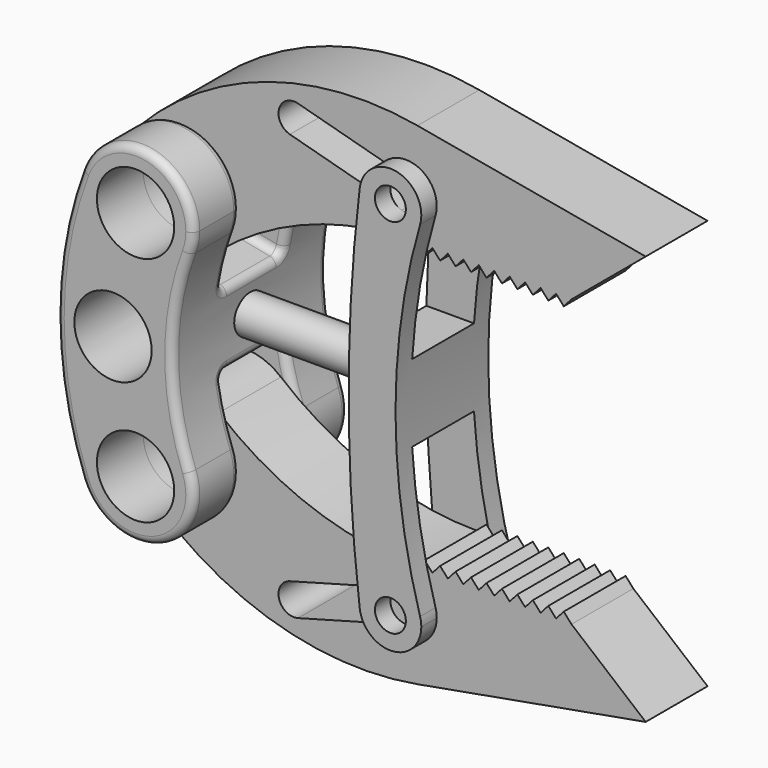
from build123d import *

# Parameters (mm, degrees)
F0_R           = 5
F2_DEPTH       = 12.5
F1_R           = 5
F3_DEPTH       = 5
F4_R           = 5
F5_DEPTH       = 25.001
F6_R           = 5
F7_DEPTH       = 5
F8_R           = 2.5
F9_DEPTH       = 60.001
F9_DEPTH_BACK  = 10.2360656985
F10_DEPTH      = 27
F10_DEPTH_BACK = 10
F11_R          = 2
F12_DEPTH      = 7.5
F14_DEPTH      = 5
F15_R          = 1


# Not quite as in the source:
# - a feature of the source that left no trace in its solid (it failed there, or was rolled back) is left out


with BuildPart() as f2:
    # F0 (on Front) → F2 (new body, symmetric)
    with BuildSketch(Plane.XZ):
        with BuildLine():
            ThreePointArc((7.0173413473, 12.3529411765), (-2.6470588235, 7.9826586527), (-7.0173413473, 17.6470588235))
            ThreePointArc((-7.0173413473, 17.6470588235), (-10.2350656985, 0), (-7.0173413473, -17.6470588235))
            ThreePointArc((-7.0173413473, -17.6470588235), (-2.6470588235, -7.9826586527), (7.0173413473, -12.3529411765))
            ThreePointArc((7.0173413473, -12.3529411765), (4.7649343015, 0), (7.0173413473, 12.3529411765))
        make_face()
        with BuildLine():
            ThreePointArc((7.5, 15), (1.3453512358, 22.3783487348), (-7.0173413473, 17.6470588235))
            ThreePointArc((-7.0173413473, 17.6470588235), (-2.6470588235, 7.9826586527), (7.0173413473, 12.3529411765))
            ThreePointArc((7.0173413473, 12.3529411765), (7.3783487348, 13.6546487642), (7.5, 15))
        make_face()
        with Locations((0, 15)):
            Circle(F0_R, mode=Mode.SUBTRACT)
        with BuildLine():
            ThreePointArc((7.0173413473, -12.3529411765), (-2.6470588235, -7.9826586527), (-7.0173413473, -17.6470588235))
            ThreePointArc((-7.0173413473, -17.6470588235), (1.3453512358, -22.3783487348), (7.5, -15))
            ThreePointArc((7.5, -15), (7.3783487348, -13.6546487642), (7.0173413473, -12.3529411765))
        make_face()
        with Locations((0, -15)):
            Circle(F0_R, mode=Mode.SUBTRACT)
    extrude(amount=F2_DEPTH, both=True)

    # F4 (on face) → F5 (cut, through all)
    with BuildSketch(Plane.XZ.offset(12.5)):
        with Locations((-2.9190075645, 0)):
            Circle(F4_R)
    extrude(amount=-F5_DEPTH, mode=Mode.SUBTRACT)

    # F6 (on Front) → F7 (cut, symmetric)
    with BuildSketch(Plane.XZ):
        with Locations((-2.9190075645, 0)):
            Circle(F6_R)
        with BuildLine():
            ThreePointArc((-7.0173413473, 17.6470588235), (-8.6192999027, 12.6081672132), (-9.6801930524, 7.4282825042))
            Line((-9.6801930524, 7.4282825042), (5.0631545713, 4.5592196216))
            ThreePointArc((5.0631545713, 4.5592196216), (5.8158548913, 8.5123444011), (7.0173413473, 12.3529411765))
            ThreePointArc((7.0173413473, 12.3529411765), (2.6470588235, 22.0173413473), (-7.0173413473, 17.6470588235))
        make_face()
        with Locations((0, 15)):
            Circle(F6_R, mode=Mode.SUBTRACT)
        with BuildLine():
            Line((5.0631545713, -4.5592196216), (-9.6801930524, -7.4282825042))
            ThreePointArc((-9.6801930524, -7.4282825042), (-8.6192999027, -12.6081672132), (-7.0173413473, -17.6470588235))
            ThreePointArc((-7.0173413473, -17.6470588235), (2.6470588235, -22.0173413473), (7.0173413473, -12.3529411765))
            ThreePointArc((7.0173413473, -12.3529411765), (5.8158548913, -8.5123444011), (5.0631545713, -4.5592196216))
        make_face()
    extrude(amount=F7_DEPTH, both=True, mode=Mode.SUBTRACT)

    # F8 (on Right) → F9 (cut, two sides)
    with BuildSketch(Plane.YZ) as f9_sk:
        Circle(F8_R)
    extrude(amount=F9_DEPTH, mode=Mode.SUBTRACT)
    extrude(f9_sk.sketch, amount=-F9_DEPTH_BACK, mode=Mode.SUBTRACT)

    # F15
    f15_edges = [f2.edges().sort_by_distance(p)[0] for p in [
        (4.764934, 12.5, 0),
        (4.764934, -12.5, 0),
        (-9.680193, 0, 7.428283),
        (-2.308519, 5, 5.993751),
        (5.063155, 0, 4.55922),
        (-2.308519, -5, 5.993751),
        (-2.308519, 5, -5.993751),
        (-9.680193, 0, -7.428283),
        (-2.308519, -5, -5.993751),
        (5.063155, 0, -4.55922),
        (5.815855, 5, 8.512344),
        (-8.6193, 5, 12.608167),
        (-10.235066, 12.5, 0),
        (-8.6193, -5, 12.608167),
        (-8.6193, 5, -12.608167),
        (-10.235066, -12.5, 0),
        (-8.6193, -5, -12.608167),
        (2.647059, 12.5, 22.017341),
        (2.647059, 12.5, -22.017341),
        (2.647059, -12.5, 22.017341),
        (2.647059, -12.5, -22.017341),
    ]]
    fillet(f15_edges, radius=F15_R)


with BuildPart() as f3:
    # F1 (on Front) → F3 (new body, symmetric)
    with BuildSketch(Plane.XZ):
        with BuildLine():
            Line((60, 26.5032651249), (30.4732648861, 31.8109871895))
            ThreePointArc((30.4732648861, 31.8109871895), (11.0839552583, 30.4999380696), (-5.3991466461, 20.2056906836))
            ThreePointArc((-5.3991466461, 20.2056906836), (-5.4923369903, 9.8927273046), (4.80020345, 9.2373576513))
            ThreePointArc((4.80020345, 9.2373576513), (16.7881276244, 16.1155217779), (30.4012885164, 18.5032651249))
            Line((30.4012885164, 18.5032651249), (31.4012885164, 17.3852311362))
            Line((31.4012885164, 17.3852311362), (32.4012885164, 18.5032651249))
            Line((32.4012885164, 18.5032651249), (33.4012885164, 17.3852311362))
            Line((33.4012885164, 17.3852311362), (34.4012885164, 18.5032651249))
            Line((34.4012885164, 18.5032651249), (35.4012885164, 17.3852311362))
            Line((35.4012885164, 17.3852311362), (36.4012885164, 18.5032651249))
            Line((36.4012885164, 18.5032651249), (37.4012885164, 17.3852311362))
            Line((37.4012885164, 17.3852311362), (38.4012885164, 18.5032651249))
            Line((38.4012885164, 18.5032651249), (39.4012885164, 17.3852311362))
            Line((39.4012885164, 17.3852311362), (40.4012885164, 18.5032651249))
            Line((40.4012885164, 18.5032651249), (41.4012885164, 17.3852311362))
            Line((41.4012885164, 17.3852311362), (42.4012885164, 18.5032651249))
            Line((42.4012885164, 18.5032651249), (43.4012885164, 17.3852311362))
            Line((43.4012885164, 17.3852311362), (44.4012885164, 18.5032651249))
            Line((44.4012885164, 18.5032651249), (45.4012885164, 17.3852311362))
            Line((45.4012885164, 17.3852311362), (46.4012885164, 18.5032651249))
            Line((46.4012885164, 18.5032651249), (47.4012885164, 17.3852311362))
            Line((47.4012885164, 17.3852311362), (48.4012885164, 18.5032651249))
            Line((48.4012885164, 18.5032651249), (49.4012885164, 17.3852311362))
            Line((49.4012885164, 17.3852311362), (50.4012885164, 18.5032651249))
            Line((50.4012885164, 18.5032651249), (60, 26.5032651249))
        make_face()
        with Locations((0, 15)):
            Circle(F1_R, mode=Mode.SUBTRACT)
        with BuildLine():
            ThreePointArc((13.9694577704, 25.4454348944), (12.5634024768, 27.899616736), (15.0175843183, 29.3056720296))
            Line((15.0175843183, 29.3056720296), (29.4934735751, 25.3751974748))
            ThreePointArc((29.4934735751, 25.3751974748), (30.5581403833, 24.6599602702), (30.9694103012, 23.4450789073))
            ThreePointArc((30.9694103012, 23.4450789073), (30.1842916641, 21.8563488251), (28.4453470272, 21.5149603397))
            Line((28.4453470272, 21.5149603397), (13.9694577704, 25.4454348944))
        make_face(mode=Mode.SUBTRACT)
    extrude(amount=F3_DEPTH, both=True)


with BuildPart() as f3b:
    # F1 (on Front) → F3, piece 2 (new body, symmetric)
    with BuildSketch(Plane.XZ):
        with BuildLine():
            ThreePointArc((4.80020345, -9.2373576513), (-5.4923369903, -9.8927273046), (-5.3991466461, -20.2056906836))
            ThreePointArc((-5.3991466461, -20.2056906836), (11.0839552583, -30.4999380696), (30.4732648861, -31.8109871895))
            Line((30.4732648861, -31.8109871895), (60, -26.5032651249))
            Line((60, -26.5032651249), (50.4012885164, -18.5032651249))
            Line((50.4012885164, -18.5032651249), (49.4012885164, -17.3852311362))
            Line((49.4012885164, -17.3852311362), (48.4012885164, -18.5032651249))
            Line((48.4012885164, -18.5032651249), (47.4012885164, -17.3852311362))
            Line((47.4012885164, -17.3852311362), (46.4012885164, -18.5032651249))
            Line((46.4012885164, -18.5032651249), (45.4012885164, -17.3852311362))
            Line((45.4012885164, -17.3852311362), (44.4012885164, -18.5032651249))
            Line((44.4012885164, -18.5032651249), (43.4012885164, -17.3852311362))
            Line((43.4012885164, -17.3852311362), (42.4012885164, -18.5032651249))
            Line((42.4012885164, -18.5032651249), (41.4012885164, -17.3852311362))
            Line((41.4012885164, -17.3852311362), (40.4012885164, -18.5032651249))
            Line((40.4012885164, -18.5032651249), (39.4012885164, -17.3852311362))
            Line((39.4012885164, -17.3852311362), (38.4012885164, -18.5032651249))
            Line((38.4012885164, -18.5032651249), (37.4012885164, -17.3852311362))
            Line((37.4012885164, -17.3852311362), (36.4012885164, -18.5032651249))
            Line((36.4012885164, -18.5032651249), (35.4012885164, -17.3852311362))
            Line((35.4012885164, -17.3852311362), (34.4012885164, -18.5032651249))
            Line((34.4012885164, -18.5032651249), (33.4012885164, -17.3852311362))
            Line((33.4012885164, -17.3852311362), (32.4012885164, -18.5032651249))
            Line((32.4012885164, -18.5032651249), (31.4012885164, -17.3852311362))
            Line((31.4012885164, -17.3852311362), (30.4012885164, -18.5032651249))
            ThreePointArc((30.4012885164, -18.5032651249), (16.7881276244, -16.1155217779), (4.80020345, -9.2373576513))
        make_face()
        with BuildLine():
            ThreePointArc((15.0175843183, -29.3056720296), (12.5634024768, -27.899616736), (13.9694577704, -25.4454348944))
            Line((13.9694577704, -25.4454348944), (28.4453470272, -21.5149603397))
            ThreePointArc((28.4453470272, -21.5149603397), (30.1842916641, -21.8563488251), (30.9694103012, -23.4450789073))
            ThreePointArc((30.9694103012, -23.4450789073), (30.5581403833, -24.6599602702), (29.4934735751, -25.3751974748))
            Line((29.4934735751, -25.3751974748), (15.0175843183, -29.3056720296))
        make_face(mode=Mode.SUBTRACT)
        with Locations((0, -15)):
            Circle(F1_R, mode=Mode.SUBTRACT)
    extrude(amount=F3_DEPTH, both=True)


with BuildPart() as f10:
    # F8 (on Right) → F10 (new body, two sides)
    with BuildSketch(Plane.YZ) as f10_sk:
        Circle(F8_R)
    extrude(amount=F10_DEPTH)
    extrude(f10_sk.sketch, amount=-F10_DEPTH_BACK)

    # F11 (on Front) → F12 (join, symmetric)
    with BuildSketch(Plane.XZ):
        with BuildLine():
            ThreePointArc((32.8104490741, 22.3286465784), (32.9294705969, 22.8812327809), (32.9694103012, 23.4450789073))
            ThreePointArc((32.9694103012, 23.4450789073), (29.2090763864, 27.4378924726), (24.9981302174, 23.9235499054))
            ThreePointArc((24.9981302174, 23.9235499054), (28.1693041486, 19.5259169886), (32.8104490741, 22.3286465784))
        make_face()
        with Locations((28.9694103012, 23.4450789073)):
            Circle(F11_R, mode=Mode.SUBTRACT)
        with BuildLine():
            ThreePointArc((32.8104490741, 22.3286465784), (28.1693041486, 19.5259169886), (24.9981302174, 23.9235499054))
            ThreePointArc((24.9981302174, 23.9235499054), (23.5621344073, 0), (24.9981302174, -23.9235499054))
            ThreePointArc((24.9981302174, -23.9235499054), (28.1693041486, -19.5259169886), (32.8104490741, -22.3286465784))
            ThreePointArc((32.8104490741, -22.3286465784), (29.6312245321, 0), (32.8104490741, 22.3286465784))
        make_face()
        with BuildLine():
            ThreePointArc((32.8104490741, -22.3286465784), (28.1693041486, -19.5259169886), (24.9981302174, -23.9235499054))
            ThreePointArc((24.9981302174, -23.9235499054), (29.2090763864, -27.4378924726), (32.9694103012, -23.4450789073))
            ThreePointArc((32.9694103012, -23.4450789073), (32.9294705969, -22.8812327809), (32.8104490741, -22.3286465784))
        make_face()
        with Locations((28.9694103012, -23.4450789073)):
            Circle(F11_R, mode=Mode.SUBTRACT)
    extrude(amount=F12_DEPTH, both=True)

    # F13 (on Front) → F14 (cut, symmetric)
    with BuildSketch(Plane.XZ):
        with BuildLine():
            ThreePointArc((24.9981302174, 23.9235499054), (24.0868591242, 14.4780713757), (23.6246441759, 5))
            Line((23.6246441759, 5), (29.7876274188, 5))
            ThreePointArc((29.7876274188, 5), (30.8213145819, 13.7476577511), (32.8104490741, 22.3286465784))
            ThreePointArc((32.8104490741, 22.3286465784), (29.7695164537, 27.3642408259), (24.9981302174, 23.9235499054))
        make_face()
        with BuildLine():
            Line((29.7876274188, -5), (23.6246441759, -5))
            ThreePointArc((23.6246441759, -5), (24.0868591242, -14.4780713757), (24.9981302174, -23.9235499054))
            ThreePointArc((24.9981302174, -23.9235499054), (29.7695164537, -27.3642408259), (32.8104490741, -22.3286465784))
            ThreePointArc((32.8104490741, -22.3286465784), (30.8213145819, -13.7476577511), (29.7876274188, -5))
        make_face()
    extrude(amount=F14_DEPTH, both=True, mode=Mode.SUBTRACT)


solid = Compound([f2.part, f3.part, f3b.part, f10.part])
